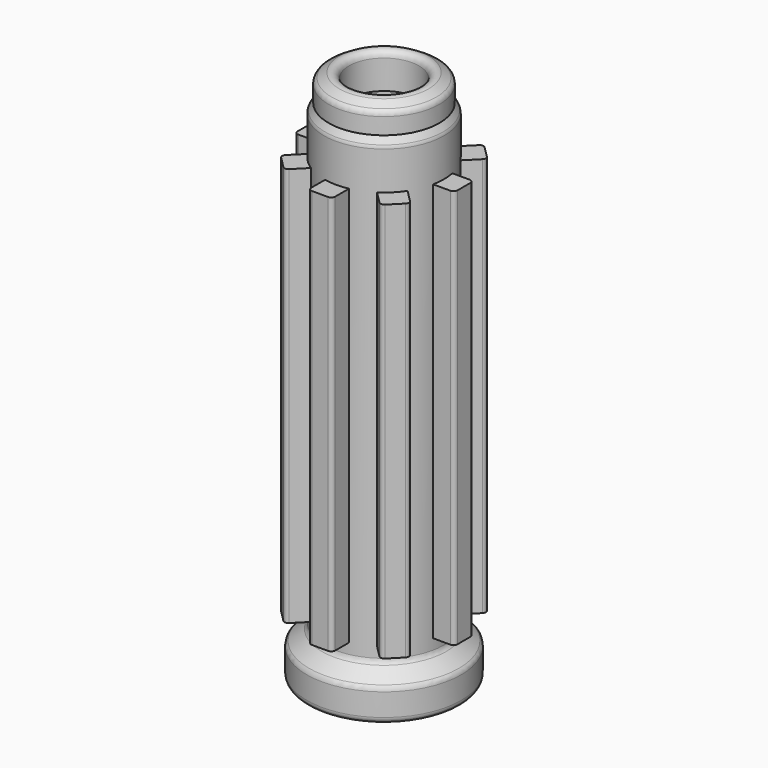
from build123d import *

# Parameters (mm, degrees)
F2_R            = 1.6
F4_W            = 6
F4_H            = 100
F5_COPIES_COUNT = 8
F6_R            = 1
F6_2_R          = 1
F6_3_R          = 1
F6_4_R          = 1
F6_5_R          = 1
F6_6_R          = 1
F6_7_R          = 1
F6_8_R          = 1


# Not quite as in the source:
# - a feature of the source that left no trace in its solid (it failed there, or was rolled back) is left out
# - a pattern or mirror of a feature is missing from the dataset's text; its kind, count and spacing are read off the source's solid


with BuildPart() as f1:
    # F0 (on Front) → F1 (revolve)
    with BuildSketch(Plane.XZ):
        with BuildLine():
            ThreePointArc((13.8452994616, 132), (11.3302729145, 133.5554082968), (8.75, 135))
            Line((8.75, 135), (8.75, 125))
            Line((8.75, 125), (10.75, 125))
            Line((10.75, 125), (10.75, 0))
            Line((10.75, 0), (19.325, 0))
            Line((19.325, 0), (19.325, 8))
            Line((19.325, 8), (15, 11.6291059048))
            Line((15, 11.6291059048), (15, 125))
            Line((15, 125), (13.8452994616, 127))
            Line((13.8452994616, 127), (13.8452994616, 132))
        make_face()
    revolve(axis=Axis((0, 0, 15.7782279773), (0, 0, -1)))

    # F2
    f2_edges = [f1.edges().sort_by_distance(p)[0] for p in [
        (-8.75, 0, 135),
        (-13.845299, 0, 132),
        (-15, 0, 125),
        (-15, 0, 11.629106),
        (-19.325, 0, 8),
        (-19.325, 0, 0),
    ]]
    fillet(f2_edges, radius=F2_R)


with BuildPart() as f5:
    # F4 (on offset) → F5 (new body, up to the next surface of F1)
    with BuildSketch(Plane.YZ.offset(20)):
        with Locations((0, 65)):
            Rectangle(F4_W, F4_H)
    extrude(until=Until.NEXT, target=f1.part, dir=(-1, 0, 0))


with BuildPart() as f5_copies_1:
    # F5_copies: instance of F5
    add(f5.part.rotate(Axis((0, 0, 0), (0, 0, 1)), 1 * 360 / F5_COPIES_COUNT))

    # F6#2
    f6_2_edges = [f5_copies_1.edges().sort_by_distance(p)[0] for p in [
        (16.263456, 12.020815, 65),
        (12.020815, 16.263456, 65),
    ]]
    fillet(f6_2_edges, radius=F6_2_R)


with BuildPart() as f5_copies_2:
    # F5_copies: instance of F5
    add(f5.part.rotate(Axis((0, 0, 0), (0, 0, 1)), 2 * 360 / F5_COPIES_COUNT))

    # F6#3
    f6_3_edges = [f5_copies_2.edges().sort_by_distance(p)[0] for p in [
        (3, 20, 65),
        (-3, 20, 65),
    ]]
    fillet(f6_3_edges, radius=F6_3_R)


with BuildPart() as f5_copies_3:
    # F5_copies: instance of F5
    add(f5.part.rotate(Axis((0, 0, 0), (0, 0, 1)), 3 * 360 / F5_COPIES_COUNT))

    # F6#4
    f6_4_edges = [f5_copies_3.edges().sort_by_distance(p)[0] for p in [
        (-12.020815, 16.263456, 65),
        (-16.263456, 12.020815, 65),
    ]]
    fillet(f6_4_edges, radius=F6_4_R)


with BuildPart() as f5_copies_4:
    # F5_copies: instance of F5
    add(f5.part.rotate(Axis((0, 0, 0), (0, 0, 1)), 4 * 360 / F5_COPIES_COUNT))

    # F6#5
    f6_5_edges = [f5_copies_4.edges().sort_by_distance(p)[0] for p in [
        (-20, 3, 65),
        (-20, -3, 65),
    ]]
    fillet(f6_5_edges, radius=F6_5_R)


with BuildPart() as f5_copies_5:
    # F5_copies: instance of F5
    add(f5.part.rotate(Axis((0, 0, 0), (0, 0, 1)), 5 * 360 / F5_COPIES_COUNT))

    # F6#6
    f6_6_edges = [f5_copies_5.edges().sort_by_distance(p)[0] for p in [
        (-16.263456, -12.020815, 65),
        (-12.020815, -16.263456, 65),
    ]]
    fillet(f6_6_edges, radius=F6_6_R)


with BuildPart() as f5_copies_6:
    # F5_copies: instance of F5
    add(f5.part.rotate(Axis((0, 0, 0), (0, 0, 1)), 6 * 360 / F5_COPIES_COUNT))

    # F6#7
    f6_7_edges = [f5_copies_6.edges().sort_by_distance(p)[0] for p in [
        (-3, -20, 65),
        (3, -20, 65),
    ]]
    fillet(f6_7_edges, radius=F6_7_R)


with BuildPart() as f5_copies_7:
    # F5_copies: instance of F5
    add(f5.part.rotate(Axis((0, 0, 0), (0, 0, 1)), 7 * 360 / F5_COPIES_COUNT))

    # F6#8
    f6_8_edges = [f5_copies_7.edges().sort_by_distance(p)[0] for p in [
        (12.020815, -16.263456, 65),
        (16.263456, -12.020815, 65),
    ]]
    fillet(f6_8_edges, radius=F6_8_R)


with BuildPart() as f5_1:
    add(f5.part)

    # F6
    f6_edges = [f5_1.edges().sort_by_distance(p)[0] for p in [
        (20, -3, 65),
        (20, 3, 65),
    ]]
    fillet(f6_edges, radius=F6_R)


solid = Compound([f1.part, f5_copies_1.part, f5_copies_2.part, f5_copies_3.part, f5_copies_4.part, f5_copies_5.part, f5_copies_6.part, f5_copies_7.part, f5_1.part])
